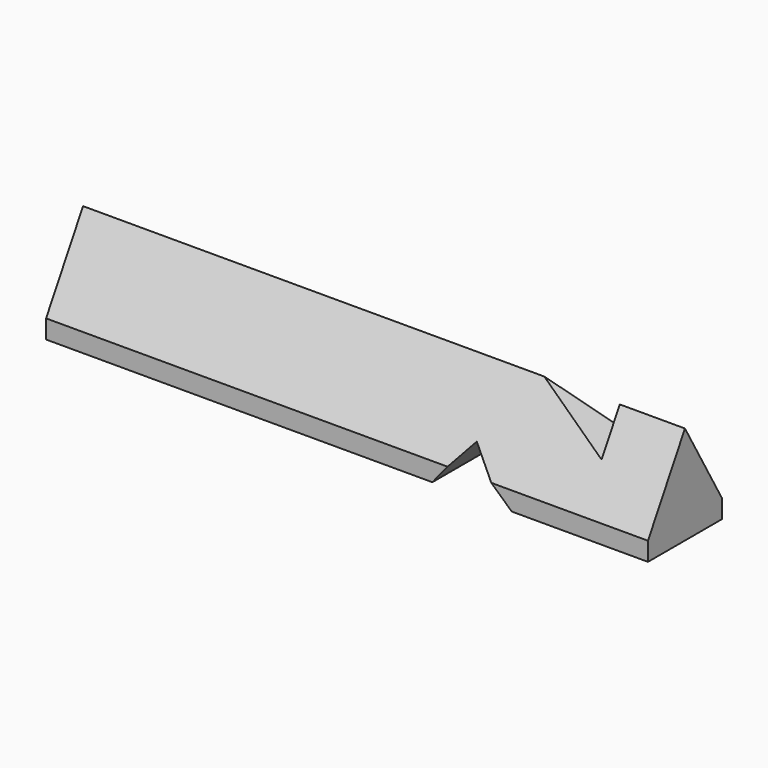
from build123d import *

# Parameters (mm, degrees)
F1_DEPTH    = 19.812
F2_T1_DEPTH = 189.0971878823
F3_T1_DEPTH = 189.0971878823
F3_T3_DEPTH = 105.0231878823


# Not quite as in the source:
# - a fillet or chamfer that OpenCascade refuses, or shapes differently, is made with other operations: its cross-section is extruded or revolved along the edge and cut away or added


with BuildPart() as f1:
    # F0 (on Front) → F1 (new body)
    with BuildSketch(Plane.XZ):
        Polygon((35.306, 9.8661940299), (33.528, 10.795), (-64.516, 10.795), (-64.516, -10.795), (18.288, -10.795), (25.5529864014, -1.905), (35.306, -10.795), align=None)
        Polygon((50.546, -10.795), (50.546, 1.905), (35.306, 9.8661940299), (35.306, -10.795), align=None)
        Polygon((64.516, -10.795), (64.516, 10.795), (50.546, 10.795), (50.546, 1.905), (50.546, -10.795), align=None)
    extrude(amount=F1_DEPTH)

    # F2: chamfer of 10.16 x 17.5976362049 on 1 edges, made by hand

    # F2_s2 → F2_t1 (cut)
    with BuildSketch(Plane.YZ.offset(-110.0425939411)):
        Polygon((-9.652, 10.795), (-19.812, -6.8026362049), (-19.812, 10.795), align=None)
    extrude(amount=F2_T1_DEPTH, mode=Mode.SUBTRACT)

    # F3: chamfer of 10.16 x 17.5976362049 on 2 edges, made by hand

    # F3_s2 → F3_t1 (cut)
    with BuildSketch(Plane.YZ.offset(-110.0425939411)):
        Polygon((0, -6.8026362049), (-10.16, 10.795), (0, 10.795), align=None)
    extrude(amount=F3_T1_DEPTH, mode=Mode.SUBTRACT)

    # F3_s4 → F3_t3 (cut)
    with BuildSketch(Plane.YZ.offset(5.0194060589)):
        Polygon((0, -6.8026362049), (-10.16, 10.795), (0, 10.795), align=None)
    extrude(amount=F3_T3_DEPTH, mode=Mode.SUBTRACT)


solid = f1.part
